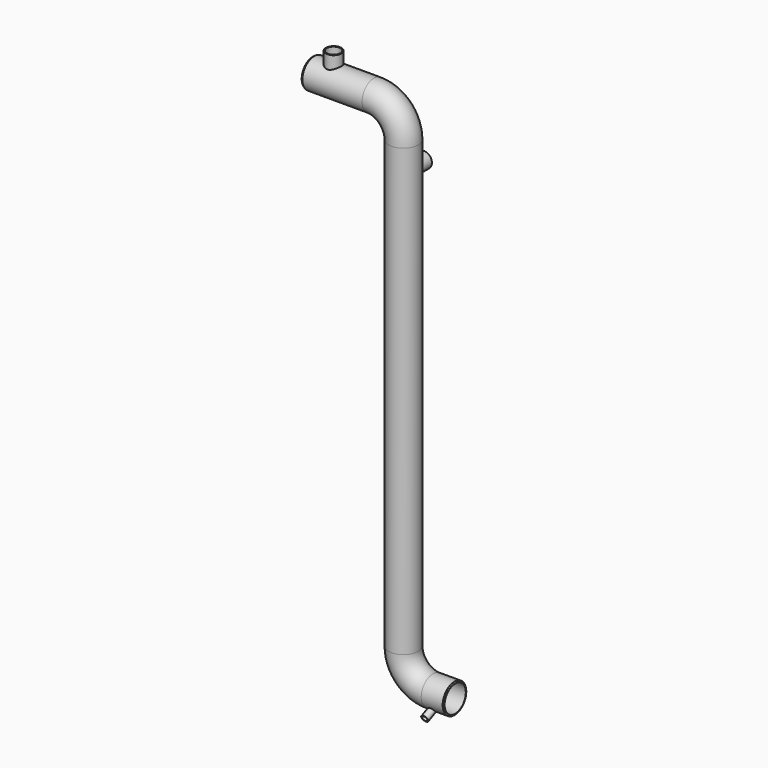
from build123d import *

# Parameters (mm, degrees)
F1_R         = 57.15
F1_R_2       = 51.15
F3_R         = 30.15
F3_R_2       = 26.25
F4_DEPTH     = 100
F5_R         = 26.25
F6_DEPTH     = 100
F7_R         = 51.15
F8_DEPTH     = 130
F10_R        = 13.35
F10_R_2      = 10.45
F11_DEPTH    = 90
F12_R        = 51.15
F13_DEPTH    = 80
F14_R        = 10.45
F15_DEPTH    = 100
F16_C1_SIZE2 = 2.8867513459
F16_C1_SIZE  = 5
F16_C2_SIZE2 = 5
F16_C2_SIZE  = 2.8867513459
F17_R        = 30.15
F18_DEPTH    = 100
F19_R        = 26.25
F20_DEPTH    = 120


with BuildPart() as f2:
    # F2: sweep along a path in F0
    with BuildLine(Plane.XZ) as f2_path:
        Line((0, 0), (235.7, 0))
        ThreePointArc((235.7, 0), (316.5223050896, -33.4776949104), (350, -114.3))
        Line((350, -114.3), (350, -1837.7))
        ThreePointArc((350, -1837.7), (383.4776949104, -1918.5223050896), (464.3, -1952))
        Line((464.3, -1952), (550, -1952))
    # F1 (on Right) → F2 (sweep)
    with BuildSketch(Plane.YZ):
        Circle(F1_R)
        Circle(F1_R_2, mode=Mode.SUBTRACT)
    sweep(path=f2_path.line)

    # F3 (on Top) → F4 (join)
    with BuildSketch(Plane.XY):
        with Locations((80, 0)):
            Circle(F3_R)
        with Locations((80, 0)):
            Circle(F3_R_2, mode=Mode.SUBTRACT)
    extrude(amount=F4_DEPTH)

    # F5 (on face) → F6 (cut)
    with BuildSketch(Plane.XY.offset(100)):
        with Locations((80, 0)):
            Circle(F5_R)
    extrude(amount=-F6_DEPTH, mode=Mode.SUBTRACT)

    # F7 (on Right) → F8 (cut)
    with BuildSketch(Plane.YZ):
        Circle(F7_R)
    extrude(amount=F8_DEPTH, mode=Mode.SUBTRACT)

    # F10 (on face) → F11 (join)
    with BuildSketch(Plane(origin=(0, -747.6593764841, -348.6392929459), x_dir=(-1, 0, 0), z_dir=(0, 0.906307787, 0.4226182617))):
        with Locations((-490, -1791.9628002955)):
            Circle(F10_R)
        with Locations((-490, -1791.9628002955)):
            Circle(F10_R_2, mode=Mode.SUBTRACT)
    extrude(amount=-F11_DEPTH)

    # F12 (on face) → F13 (cut)
    with BuildSketch(Plane.YZ.offset(550)):
        with Locations((0, -1952)):
            Circle(F12_R)
    extrude(amount=-F13_DEPTH, mode=Mode.SUBTRACT)

    # F14 (on face) → F15 (cut)
    with BuildSketch(Plane(origin=(0, -829.2270773174, -386.6749365026), x_dir=(1, 0, 0), z_dir=(0, -0.906307787, -0.4226182617))):
        with Locations((490, -1791.9628002955)):
            Circle(F14_R)
    extrude(amount=-F15_DEPTH, mode=Mode.SUBTRACT)

    # F16: chamfer of 5 x 2.8867513459 on 2 edges, made by hand

    # F16_c1
    f16_c1_edges = [f2.edges().sort_by_distance(p)[0] for p in [
        (0, -57.15, 0),
    ]]
    f16_c1_side = f2.faces().sort_by_distance((0.0577350269, -57.15, 0))[0]
    chamfer(f16_c1_edges, length=F16_C1_SIZE, length2=F16_C1_SIZE2, reference=f16_c1_side)

    # F16_c2
    f16_c2_edges = [f2.edges().sort_by_distance(p)[0] for p in [
        (550, -57.15, -1952),
    ]]
    f16_c2_side = f2.faces().sort_by_distance((549.9422649731, -57.15, -1952))[0]
    chamfer(f16_c2_edges, length=F16_C2_SIZE, length2=F16_C2_SIZE2, reference=f16_c2_side)

    # F17 (on Front) → F18 (join)
    with BuildSketch(Plane.XZ):
        with Locations((349.85, -224.3)):
            Circle(F17_R)
    extrude(amount=-F18_DEPTH)

    # F19 (on face) → F20 (cut)
    with BuildSketch(Plane(origin=(0, 100, 0), x_dir=(-1, 0, 0), z_dir=(0, 1, 0))):
        with Locations((-349.85, -224.3)):
            Circle(F19_R)
    extrude(amount=-F20_DEPTH, mode=Mode.SUBTRACT)


solid = f2.part
